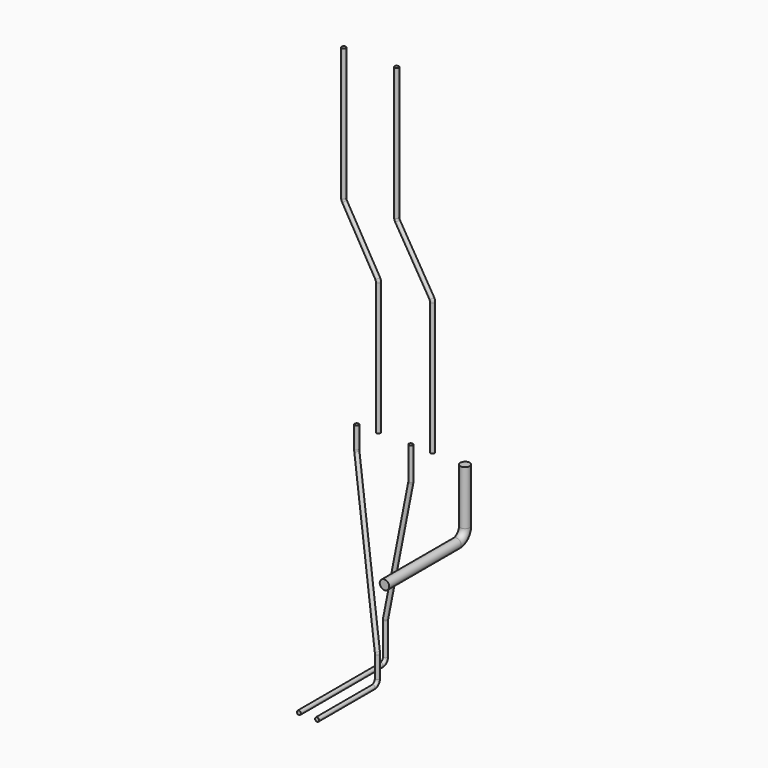
from build123d import *

# Parameters (mm, degrees)
F0_R   = 4.7625
F0_R_2 = 11.1125


# Not quite as in the source:
# - a feature names something its author has since deleted; it is built from what else it names


with BuildPart() as f2:
    # F2: sweep along a path in F1
    with BuildLine(Plane.XZ) as f2_path:
        Line((0, 0), (0, 310.7981686801))
        ThreePointArc((0, 310.7981686801), (-0.4630874045, 314.1963991211), (-1.8185779732, 317.3468062999))
        Line((-1.8185779732, 317.3468062999), (-82.2554220268, 451.0031937001))
        ThreePointArc((-82.2554220268, 451.0031937001), (-83.6109125955, 454.1536008789), (-84.074, 457.5518313199))
        Line((-84.074, 457.5518313199), (-84.074, 768.35))
    # F0 (on Top) → F2 (sweep)
    with BuildSketch(Plane.XY):
        Circle(F0_R)
    sweep(path=f2_path.line)


with BuildPart() as f3:
    # F3: sweep along a path in F1
    with BuildLine(Plane.XZ) as f3_path:
        Line((-127, 0), (-127, 310.7981686801))
        ThreePointArc((-127, 310.7981686801), (-127.4371711548, 314.1016560366), (-128.7185871991, 317.1777119942))
        Line((-128.7185871991, 317.1777119942), (-206.5614128009, 451.1722880058))
        ThreePointArc((-206.5614128009, 451.1722880058), (-207.8428288452, 454.2483439634), (-208.28, 457.5518313199))
        Line((-208.28, 457.5518313199), (-208.28, 768.35))
    # F0 (on Top) → F3 (sweep)
    with BuildSketch(Plane.XY):
        with Locations((-127, 0)):
            Circle(F0_R)
    sweep(path=f3_path.line)


with BuildPart() as f7:
    # F7: sweep along a path in F6
    with BuildLine(Plane.YZ.offset(76.2)) as f7_path:
        Line((0, 0), (0, -127))
        ThreePointArc((0, -127), (-7.4394877579, -144.9605122421), (-25.4, -152.4))
        Line((-25.4, -152.4), (-236.22, -152.4))
    # F0 (on Top) → F7 (sweep)
    with BuildSketch(Plane.XY):
        with Locations((76.2, 0)):
            Circle(F0_R_2)
    sweep(path=f7_path.line)


with BuildPart() as f9:
    # F9: sweep along a path in F1, F8
    with BuildLine(Plane.XZ) as f9_path:
        Line((-50.8, 0), (-50.8, -76.2))
        ThreePointArc((-50.8, -76.2), (-50.8597738423, -77.4307244538), (-51.0385327057, -78.6498638479))
        Line((-51.0385327057, -78.6498638479), (-109.9974672943, -378.5501361521))
        ThreePointArc((-109.9974672943, -378.5501361521), (-110.1762261577, -379.7692755462), (-110.236, -381))
        Line((-110.236, -381), (-110.236, -457.2))
    with BuildLine(Plane.YZ.offset(-110.236)) as f9_path_2:
        ThreePointArc((0, -457.2), (-3.7197438789, -466.1802561211), (-12.7, -469.9))
        Line((-12.7, -469.9), (-254, -469.9))
    # F0 (on Top) → F9 (sweep)
    with BuildSketch(Plane.XY):
        with Locations((-50.8, 0)):
            Circle(F0_R)
    sweep(path=f9_path.line + f9_path_2.line)


with BuildPart() as f14:
    # F14: sweep along a path in F11, F13
    with BuildLine(Plane(origin=(-58.4944092583, -83.5386739879, 0), x_dir=(-0.8191520443, 0.5735764364, 0), z_dir=(0.5735764364, 0.8191520443, 0))) as f14_path:
        Line((145.6452334746, 0), (145.6452334746, -50.8))
        ThreePointArc((145.6452334746, -50.8), (145.4327889753, -53.1132136986), (144.802562984, -55.3490369207))
        Line((144.802562984, -55.3490369207), (11.8679039652, -401.8509630793))
        ThreePointArc((11.8679039652, -401.8509630793), (11.2376779738, -404.0867863014), (11.0252334746, -406.4))
        Line((11.0252334746, -406.4), (11.0252334746, -457.2))
    with BuildLine(Plane.YZ.offset(-67.5257517978)) as f14_path_2:
        ThreePointArc((-77.2148598616, -457.2), (-80.9346037405, -466.1802561211), (-89.9148598616, -469.9))
        Line((-89.9148598616, -469.9), (-254, -469.9))
    # F0 (on Top) → F14 (sweep)
    with BuildSketch(Plane.XY):
        with Locations((-177.8, 0)):
            Circle(F0_R)
    sweep(path=f14_path.line + f14_path_2.line)


solid = Compound([f2.part, f3.part, f7.part, f9.part, f14.part])
